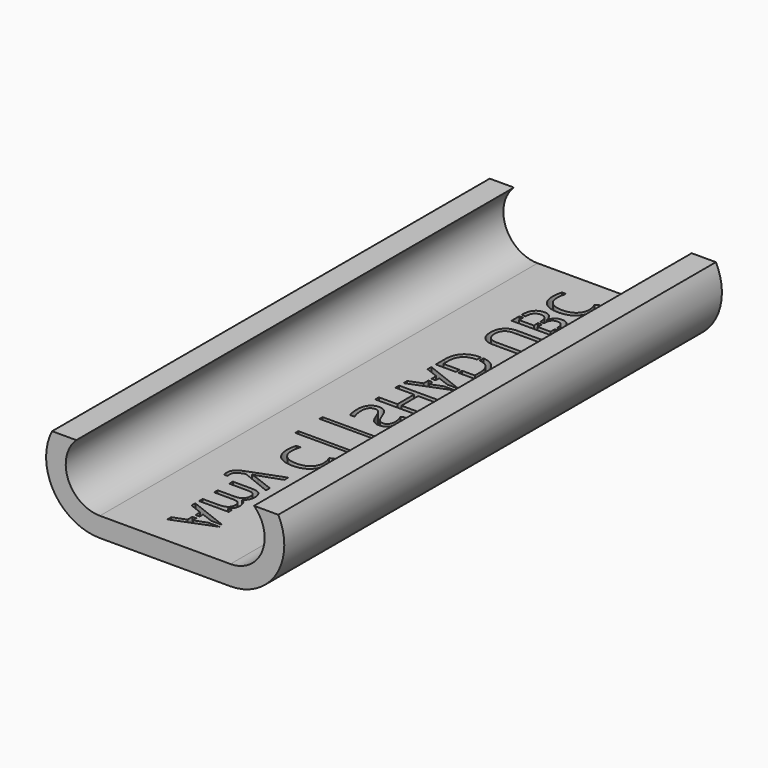
from build123d import *

# Parameters (mm, degrees)
F1_DEPTH     = 55.88
F3_DEPTH     = 55.88
F4_TEXT_SIZE = 5.6384731448
F5_DEPTH     = 12.7
F6_W         = 2.7619708295
F6_H         = 0.3930022432
F6_H_2       = 0.3938121087
F7_DEPTH     = 2.0066


# Not quite as in the source:
# - Text() gives the source's letters only with a copy of the font that has no kerning and outlines rounded to 1/6400 em; it was checked with that copy


with BuildPart() as f1:
    # F0 (on Front) → F1 (new body)
    with BuildSketch(Plane.XZ):
        with BuildLine():
            Line((6.9708472332, 5.5118), (-6.3641527668, 5.5118))
            ThreePointArc((-6.3641527668, 5.5118), (-11.8632527668, 0.0127), (-6.3641527668, -5.4864))
            Line((-6.3641527668, -5.4864), (6.9708472332, -5.4864))
            ThreePointArc((6.9708472332, -5.4864), (12.4699472332, 0.0127), (6.9708472332, 5.5118))
        make_face()
        with BuildLine():
            ThreePointArc((-6.3641527668, -3.4798), (-9.8566527668, 0.0127), (-6.3641527668, 3.5052))
            Line((-6.3641527668, 3.5052), (6.9708472332, 3.5052))
            ThreePointArc((6.9708472332, 3.5052), (10.4633472332, 0.0127), (6.9708472332, -3.4798))
            Line((6.9708472332, -3.4798), (-6.3641527668, -3.4798))
        make_face(mode=Mode.SUBTRACT)
    extrude(amount=F1_DEPTH)

    # F2 (on face) → F3 (cut)
    with BuildSketch(Plane.XZ.offset(55.88)):
        with BuildLine():
            Line((17.4389537424, 10.6313627753), (-14.7017380223, 10.6313627753))
            Line((-14.7017380223, 10.6313627753), (-14.7017380223, 2.54))
            Line((-14.7017380223, 2.54), (-11.2480912922, 2.54))
            ThreePointArc((-11.2480912922, 2.54), (-9.2226685862, 4.7104641618), (-6.3641527668, 5.5118))
            Line((-6.3641527668, 5.5118), (6.9708472332, 5.5118))
            ThreePointArc((6.9708472332, 5.5118), (9.8293630527, 4.7104641618), (11.8547857586, 2.54))
            Line((11.8547857586, 2.54), (17.4389537424, 2.54))
            Line((17.4389537424, 2.54), (17.4389537424, 10.6313627753))
        make_face()
        with BuildLine():
            ThreePointArc((-6.3641527668, 5.5118), (-9.2226685862, 4.7104641618), (-11.2480912922, 2.54))
            Line((-11.2480912922, 2.54), (-8.7746114285, 2.54))
            ThreePointArc((-8.7746114285, 2.54), (-7.6624133338, 3.2549331424), (-6.3641527668, 3.5052))
            Line((-6.3641527668, 3.5052), (6.9708472332, 3.5052))
            ThreePointArc((6.9708472332, 3.5052), (8.2691078003, 3.2549331424), (9.381305895, 2.54))
            Line((9.381305895, 2.54), (11.8547857586, 2.54))
            ThreePointArc((11.8547857586, 2.54), (9.8293630527, 4.7104641618), (6.9708472332, 5.5118))
            Line((6.9708472332, 5.5118), (-6.3641527668, 5.5118))
        make_face()
    extrude(amount=-F3_DEPTH, mode=Mode.SUBTRACT)

    # F4 (on face) → F5 (cut)
    with BuildSketch(Plane(origin=(0, 0, -5.4864), x_dir=(1, 0, 0), z_dir=(0, 0, -1))):
        with Locations(Location((-1.778, 52.9994300491), (0, 0, -90))):
            Text('Amy C||SHAD UBC', F4_TEXT_SIZE, font='Open Sans', text_align=(TextAlign.LEFT, TextAlign.BOTTOM))
    extrude(amount=-F5_DEPTH, mode=Mode.SUBTRACT)

    # F6 (on face) → F7 (join)
    with BuildSketch(Plane(origin=(0, 0, -5.4864), x_dir=(1, 0, 0), z_dir=(0, 0, -1))):
        with Locations((0.8830950209, 51.2118222869)):
            Rectangle(F6_W, F6_H)
        with Locations((0.8830950209, 21.0684923269)):
            Rectangle(F6_W, F6_H_2)
        with BuildLine():
            Line((0.5340296775, 15.5329288918), (0.5340296775, 18.7351335575))
            Line((0.5340296775, 18.7351335575), (0.2729946064, 18.7351335575))
            Line((0.2729946064, 18.7351335575), (0.2729946064, 15.5220848765))
            add(Edge.make_bspline(
                [(0.2729946064, 15.5220848765), (0.4078231201, 15.5220848765), (0.5340296775, 15.5329288918)],
                knots=[2, 2, 2, 2.1353124009, 2.1353124009, 2.1353124009], degree=2))
        make_face()
        with BuildLine():
            Line((2.2473412185, 7.9171942225), (2.2473412185, 8.0623272806))
            Line((2.2473412185, 8.0623272806), (-1.778, 8.0623272806))
            Line((-1.778, 8.0623272806), (-1.778, 7.7754692174))
            Line((-1.778, 7.7754692174), (2.2453671566, 7.7754692174))
            add(Edge.make_bspline(
                [(2.2453671566, 7.7754692174), (2.2473412185, 7.8445082528), (2.2473412185, 7.9171942225)],
                knots=[4.753618109, 4.753618109, 4.753618109, 4.8845208845, 4.8845208845, 4.8845208845], degree=2))
        make_face()
    extrude(amount=-F7_DEPTH)


solid = f1.part
